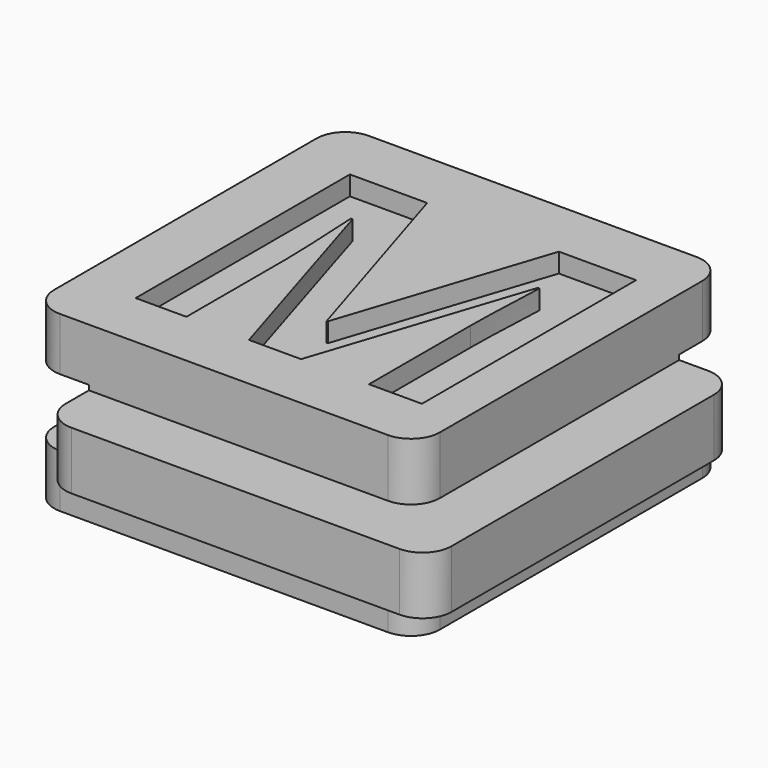
from build123d import *

# Parameters (mm, degrees)
F0_W         = 14
F0_H         = 3
F0_W_2       = 3
F1_DEPTH     = 20
F2_DEPTH     = 3
F3_W         = 3
F3_H         = 3
F4_DEPTH     = 100
F5_W         = 3
F5_H         = 3.5
F6_DEPTH     = 100
F7_R         = 1.5
F8_TEXT_SIZE = 19.4444444444
F9_DEPTH     = 1


# Not quite as in the source:
# - Text() gives the source's letters only with a copy of the font that has no kerning and outlines rounded to 1/6400 em; it was checked with that copy


with BuildPart() as f1:
    # F0 (on Front) → F1 (new body)
    with BuildSketch(Plane.XZ):
        Polygon((10, 1.5), (10, 4.5), (-10, 4.5), (-10, 1.5), (-7, 1.5), (7, 1.5), align=None)
        Rectangle(F0_W, F0_H)
        with Locations((11.5, 0)):
            Rectangle(F0_W_2, F0_H)
        with Locations((8.5, 0)):
            Rectangle(F0_W_2, F0_H)
        with Locations((-8.5, 0)):
            Rectangle(F0_W_2, F0_H)
        Polygon((10, -4.5), (10, -1.5), (7, -1.5), (-7, -1.5), (-10, -1.5), (-10, -4.5), align=None)
    extrude(amount=-F1_DEPTH)

    # F0 (on Front) → F2 (join)
    with BuildSketch(Plane.XZ):
        with Locations((-8.5, 0)):
            Rectangle(F0_W_2, F0_H)
        Rectangle(F0_W, F0_H)
        with Locations((8.5, 0)):
            Rectangle(F0_W_2, F0_H)
        with Locations((11.5, 0)):
            Rectangle(F0_W_2, F0_H)
    extrude(amount=F2_DEPTH)

    # F3 (on face) → F4 (cut)
    with BuildSketch(Plane.YZ.offset(13)):
        Polygon((23, -1.75), (23, 1.75), (17, 1.75), (17, 1.5), (20, 1.5), (20, -1.5), (17, -1.5), (17, -1.75), align=None)
        with Locations((18.5, 0)):
            Rectangle(F3_W, F3_H)
    extrude(amount=-F4_DEPTH, mode=Mode.SUBTRACT)

    # F5 (on face) → F6 (cut)
    with BuildSketch(Plane(origin=(0, 17, 0), x_dir=(-1, 0, 0), z_dir=(0, 1, 0))):
        with Locations((11.5, 0)):
            Rectangle(F5_W, F5_H)
        with Locations((8.5, 0)):
            Rectangle(F5_W, F5_H)
    extrude(amount=-F6_DEPTH, mode=Mode.SUBTRACT)

    # F7
    f7_edges = [f1.edges().sort_by_distance(p)[0] for p in [
        (-7, -3, 0),
        (13, -3, 0),
        (10, 0, 3),
        (10, 0, -3),
        (-10, 0, -3.125),
        (-10, 0, 3.125),
        (-7, 17, 0),
        (-10, 20, 3.125),
        (-10, 20, -3.125),
        (13, 17, 0),
        (10, 20, 3.125),
        (10, 20, -3.125),
    ]]
    fillet(f7_edges, radius=F7_R)

    # F8 (on face) → F9 (cut)
    with BuildSketch(Plane.XY.offset(4.5)):
        with Locations((-8.7207975495, 3)):
            Text('M', F8_TEXT_SIZE, font='Open Sans', font_style=FontStyle.BOLD, text_align=(TextAlign.LEFT, TextAlign.BOTTOM))
    extrude(amount=-F9_DEPTH, mode=Mode.SUBTRACT)


solid = f1.part
